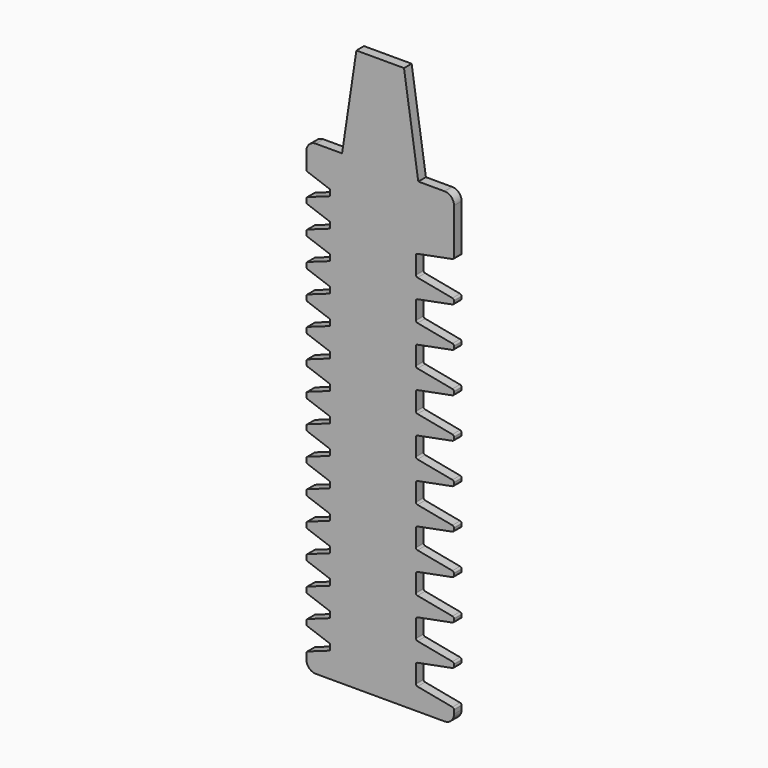
from build123d import *

# Parameters (mm, degrees)
F1_DEPTH  = 0.635
F2_R      = 1.27
F4_DEPTH  = 12.7
F6_DEPTH  = 12.7
F8_DEPTH  = 0.635
F11_DEPTH = 12.7


with BuildPart() as f1:
    # F0 (on Front) → F1 (new body, symmetric)
    with BuildSketch(Plane.XZ):
        Polygon((-9.8425, -12.7), (-9.8425, -62.23), (0, -62.23), (9.8425, -62.23), (9.8425, -12.7), (9.8425, 0), (3.175, 0), (0, 0), (-3.175, 0), (-9.8425, 0), align=None)
        Polygon((-3.175, 12.7), (-3.175, 0), (0, 0), (3.175, 0), (3.175, 12.7), (0, 12.7), align=None)
    extrude(amount=F1_DEPTH, both=True)

    # F2
    f2_edges = [f1.edges().sort_by_distance(p)[0] for p in [
        (9.8425, 0, -62.23),
        (-9.8425, 0, -62.23),
        (-9.8425, 0, 0),
        (9.8425, 0, 0),
    ]]
    fillet(f2_edges, radius=F2_R)

    # F3 (on Front) → F4 (cut, symmetric)
    with BuildSketch(Plane.XZ):
        with BuildLine():
            Line((9.8425, -57.9145550728), (9.8425, -55.3745550728))
            ThreePointArc((9.8425, -55.3745550728), (9.7843008142, -55.536351368), (9.6363736917, -55.6240026818))
            Line((9.6363736917, -55.6240026818), (4.9686263083, -56.5198312683))
            ThreePointArc((4.9686263083, -56.5198312683), (4.8206991858, -56.607482582), (4.7625, -56.7692788773))
            Line((4.7625, -56.7692788773), (4.7625, -57.9145550728))
            Line((4.7625, -57.9145550728), (9.8425, -57.9145550728))
        make_face()
        with BuildLine():
            Line((9.8425, -60.4545550728), (9.8425, -57.9145550728))
            Line((9.8425, -57.9145550728), (4.7625, -57.9145550728))
            Line((4.7625, -57.9145550728), (4.7625, -59.0598312683))
            ThreePointArc((4.7625, -59.0598312683), (4.8206991858, -59.2216275635), (4.9686263083, -59.3092788773))
            Line((4.9686263083, -59.3092788773), (9.6363736917, -60.2051074638))
            ThreePointArc((9.6363736917, -60.2051074638), (9.7843008142, -60.2927587775), (9.8425, -60.4545550728))
        make_face()
    extrude(amount=F4_DEPTH, both=True, mode=Mode.SUBTRACT)

    # F5 (on Front) → F6 (cut, symmetric)
    with BuildSketch(Plane.XZ):
        with BuildLine():
            Line((9.8425, -57.9145550728), (9.8425, -55.3745550728))
            ThreePointArc((9.8425, -55.3745550728), (9.7843008142, -55.536351368), (9.6363736917, -55.6240026818))
            Line((9.6363736917, -55.6240026818), (4.9686263083, -56.5198312683))
            ThreePointArc((4.9686263083, -56.5198312683), (4.8206991858, -56.607482582), (4.7625, -56.7692788773))
            Line((4.7625, -56.7692788773), (4.7625, -57.9145550728))
            Line((4.7625, -57.9145550728), (4.7625, -59.0598312683))
            ThreePointArc((4.7625, -59.0598312683), (4.8206991858, -59.2216275635), (4.9686263083, -59.3092788773))
            Line((4.9686263083, -59.3092788773), (9.6363736917, -60.2051074638))
            ThreePointArc((9.6363736917, -60.2051074638), (9.7843008142, -60.2927587775), (9.8425, -60.4545550728))
            Line((9.8425, -60.4545550728), (9.8425, -57.9145550728))
        make_face()
        with BuildLine():
            Line((9.6363736917, -50.2900026818), (4.9686263083, -51.1858312683))
            ThreePointArc((4.9686263083, -51.1858312683), (4.8206991858, -51.273482582), (4.7625, -51.4352788773))
            Line((4.7625, -51.4352788773), (4.7625, -52.5805550728))
            Line((4.7625, -52.5805550728), (4.7625, -53.7258312683))
            ThreePointArc((4.7625, -53.7258312683), (4.8206991858, -53.8876275635), (4.9686263083, -53.9752788773))
            Line((4.9686263083, -53.9752788773), (9.6363736917, -54.8711074638))
            ThreePointArc((9.6363736917, -54.8711074638), (9.7843008142, -54.9587587775), (9.8425, -55.1205550728))
            Line((9.8425, -55.1205550728), (9.8425, -52.5805550728))
            Line((9.8425, -52.5805550728), (9.8425, -50.0405550728))
            ThreePointArc((9.8425, -50.0405550728), (9.7843008142, -50.202351368), (9.6363736917, -50.2900026818))
        make_face()
        with BuildLine():
            Line((9.6363736917, -44.9560026818), (4.9686263083, -45.8518312683))
            ThreePointArc((4.9686263083, -45.8518312683), (4.8206991858, -45.939482582), (4.7625, -46.1012788773))
            Line((4.7625, -46.1012788773), (4.7625, -47.2465550728))
            Line((4.7625, -47.2465550728), (4.7625, -48.3918312683))
            ThreePointArc((4.7625, -48.3918312683), (4.8206991858, -48.5536275635), (4.9686263083, -48.6412788773))
            Line((4.9686263083, -48.6412788773), (9.6363736917, -49.5371074638))
            ThreePointArc((9.6363736917, -49.5371074638), (9.7843008142, -49.6247587775), (9.8425, -49.7865550728))
            Line((9.8425, -49.7865550728), (9.8425, -47.2465550728))
            Line((9.8425, -47.2465550728), (9.8425, -44.7065550728))
            ThreePointArc((9.8425, -44.7065550728), (9.7843008142, -44.868351368), (9.6363736917, -44.9560026818))
        make_face()
        with BuildLine():
            Line((9.6363736917, -39.6220026818), (4.9686263083, -40.5178312683))
            ThreePointArc((4.9686263083, -40.5178312683), (4.8206991858, -40.605482582), (4.7625, -40.7672788773))
            Line((4.7625, -40.7672788773), (4.7625, -41.9125550728))
            Line((4.7625, -41.9125550728), (4.7625, -43.0578312683))
            ThreePointArc((4.7625, -43.0578312683), (4.8206991858, -43.2196275635), (4.9686263083, -43.3072788773))
            Line((4.9686263083, -43.3072788773), (9.6363736917, -44.2031074638))
            ThreePointArc((9.6363736917, -44.2031074638), (9.7843008142, -44.2907587775), (9.8425, -44.4525550728))
            Line((9.8425, -44.4525550728), (9.8425, -41.9125550728))
            Line((9.8425, -41.9125550728), (9.8425, -39.3725550728))
            ThreePointArc((9.8425, -39.3725550728), (9.7843008142, -39.534351368), (9.6363736917, -39.6220026818))
        make_face()
        with BuildLine():
            Line((9.6363736917, -34.2880026818), (4.9686263083, -35.1838312683))
            ThreePointArc((4.9686263083, -35.1838312683), (4.8206991858, -35.271482582), (4.7625, -35.4332788773))
            Line((4.7625, -35.4332788773), (4.7625, -36.5785550728))
            Line((4.7625, -36.5785550728), (4.7625, -37.7238312683))
            ThreePointArc((4.7625, -37.7238312683), (4.8206991858, -37.8856275635), (4.9686263083, -37.9732788773))
            Line((4.9686263083, -37.9732788773), (9.6363736917, -38.8691074638))
            ThreePointArc((9.6363736917, -38.8691074638), (9.7843008142, -38.9567587775), (9.8425, -39.1185550728))
            Line((9.8425, -39.1185550728), (9.8425, -36.5785550728))
            Line((9.8425, -36.5785550728), (9.8425, -34.0385550728))
            ThreePointArc((9.8425, -34.0385550728), (9.7843008142, -34.200351368), (9.6363736917, -34.2880026818))
        make_face()
        with BuildLine():
            Line((9.6363736917, -28.9540026818), (4.9686263083, -29.8498312683))
            ThreePointArc((4.9686263083, -29.8498312683), (4.8206991858, -29.937482582), (4.7625, -30.0992788773))
            Line((4.7625, -30.0992788773), (4.7625, -31.2445550728))
            Line((4.7625, -31.2445550728), (4.7625, -32.3898312683))
            ThreePointArc((4.7625, -32.3898312683), (4.8206991858, -32.5516275635), (4.9686263083, -32.6392788773))
            Line((4.9686263083, -32.6392788773), (9.6363736917, -33.5351074638))
            ThreePointArc((9.6363736917, -33.5351074638), (9.7843008142, -33.6227587775), (9.8425, -33.7845550728))
            Line((9.8425, -33.7845550728), (9.8425, -31.2445550728))
            Line((9.8425, -31.2445550728), (9.8425, -28.7045550728))
            ThreePointArc((9.8425, -28.7045550728), (9.7843008142, -28.866351368), (9.6363736917, -28.9540026818))
        make_face()
        with BuildLine():
            Line((9.6363736917, -23.6200026818), (4.9686263083, -24.5158312683))
            ThreePointArc((4.9686263083, -24.5158312683), (4.8206991858, -24.603482582), (4.7625, -24.7652788773))
            Line((4.7625, -24.7652788773), (4.7625, -25.9105550728))
            Line((4.7625, -25.9105550728), (4.7625, -27.0558312683))
            ThreePointArc((4.7625, -27.0558312683), (4.8206991858, -27.2176275635), (4.9686263083, -27.3052788773))
            Line((4.9686263083, -27.3052788773), (9.6363736917, -28.2011074638))
            ThreePointArc((9.6363736917, -28.2011074638), (9.7843008142, -28.2887587775), (9.8425, -28.4505550728))
            Line((9.8425, -28.4505550728), (9.8425, -25.9105550728))
            Line((9.8425, -25.9105550728), (9.8425, -23.3705550728))
            ThreePointArc((9.8425, -23.3705550728), (9.7843008142, -23.532351368), (9.6363736917, -23.6200026818))
        make_face()
        with BuildLine():
            Line((9.6363736917, -18.2860026818), (4.9686263083, -19.1818312683))
            ThreePointArc((4.9686263083, -19.1818312683), (4.8206991858, -19.269482582), (4.7625, -19.4312788773))
            Line((4.7625, -19.4312788773), (4.7625, -20.5765550728))
            Line((4.7625, -20.5765550728), (4.7625, -21.7218312683))
            ThreePointArc((4.7625, -21.7218312683), (4.8206991858, -21.8836275635), (4.9686263083, -21.9712788773))
            Line((4.9686263083, -21.9712788773), (9.6363736917, -22.8671074638))
            ThreePointArc((9.6363736917, -22.8671074638), (9.7843008142, -22.9547587775), (9.8425, -23.1165550728))
            Line((9.8425, -23.1165550728), (9.8425, -20.5765550728))
            Line((9.8425, -20.5765550728), (9.8425, -18.0365550728))
            ThreePointArc((9.8425, -18.0365550728), (9.7843008142, -18.198351368), (9.6363736917, -18.2860026818))
        make_face()
        with BuildLine():
            Line((9.6363736917, -12.9520026818), (4.9686263083, -13.8478312683))
            ThreePointArc((4.9686263083, -13.8478312683), (4.8206991858, -13.935482582), (4.7625, -14.0972788773))
            Line((4.7625, -14.0972788773), (4.7625, -15.2425550728))
            Line((4.7625, -15.2425550728), (4.7625, -16.3878312683))
            ThreePointArc((4.7625, -16.3878312683), (4.8206991858, -16.5496275635), (4.9686263083, -16.6372788773))
            Line((4.9686263083, -16.6372788773), (9.6363736917, -17.5331074638))
            ThreePointArc((9.6363736917, -17.5331074638), (9.7843008142, -17.6207587775), (9.8425, -17.7825550728))
            Line((9.8425, -17.7825550728), (9.8425, -15.2425550728))
            Line((9.8425, -15.2425550728), (9.8425, -12.7025550728))
            ThreePointArc((9.8425, -12.7025550728), (9.7843008142, -12.864351368), (9.6363736917, -12.9520026818))
        make_face()
        with BuildLine():
            Line((9.6363736917, -7.6180026818), (4.9686263083, -8.5138312683))
            ThreePointArc((4.9686263083, -8.5138312683), (4.8206991858, -8.601482582), (4.7625, -8.7632788773))
            Line((4.7625, -8.7632788773), (4.7625, -9.9085550728))
            Line((4.7625, -9.9085550728), (4.7625, -11.0538312683))
            ThreePointArc((4.7625, -11.0538312683), (4.8206991858, -11.2156275635), (4.9686263083, -11.3032788773))
            Line((4.9686263083, -11.3032788773), (9.6363736917, -12.1991074638))
            ThreePointArc((9.6363736917, -12.1991074638), (9.7843008142, -12.2867587775), (9.8425, -12.4485550728))
            Line((9.8425, -12.4485550728), (9.8425, -9.9085550728))
            Line((9.8425, -9.9085550728), (9.8425, -7.3685550728))
            ThreePointArc((9.8425, -7.3685550728), (9.7843008142, -7.530351368), (9.6363736917, -7.6180026818))
        make_face()
    extrude(amount=F6_DEPTH, both=True, mode=Mode.SUBTRACT)

    # F7 (on Front) → F8 (join, symmetric)
    with BuildSketch(Plane.XZ):
        Polygon((-3.175, 12.7), (-5.08, 0), (0, 0), (5.08, 0), (3.175, 12.7), align=None)
    extrude(amount=F8_DEPTH, both=True)

    # F10 (on Front) → F11 (cut, symmetric)
    with BuildSketch(Plane.XZ):
        with BuildLine():
            Line((-9.8425, -56.769), (-9.8425, -60.198))
            ThreePointArc((-9.8425, -60.198), (-9.7961774075, -60.0517601476), (-9.6741055557, -59.9588605243))
            Line((-9.6741055557, -59.9588605243), (-6.7943923967, -58.928))
            ThreePointArc((-6.7943923967, -58.928), (-6.7024060494, -58.8579961712), (-6.6675, -58.7477982045))
            Line((-6.6675, -58.7477982045), (-6.6675, -58.2192017955))
            ThreePointArc((-6.6675, -58.2192017955), (-6.7024060494, -58.1090038288), (-6.7943923967, -58.039))
            Line((-6.7943923967, -58.039), (-9.6741055557, -57.0081394757))
            ThreePointArc((-9.6741055557, -57.0081394757), (-9.7961774075, -56.9152398524), (-9.8425, -56.769))
        make_face()
        with BuildLine():
            Line((-9.8425, -52.959), (-9.8425, -56.388))
            ThreePointArc((-9.8425, -56.388), (-9.7961774075, -56.2417601476), (-9.6741055557, -56.1488605243))
            Line((-9.6741055557, -56.1488605243), (-6.7943923967, -55.118))
            ThreePointArc((-6.7943923967, -55.118), (-6.7024060494, -55.0479961712), (-6.6675, -54.9377982045))
            Line((-6.6675, -54.9377982045), (-6.6675, -54.4092017955))
            ThreePointArc((-6.6675, -54.4092017955), (-6.7024060494, -54.2990038288), (-6.7943923967, -54.229))
            Line((-6.7943923967, -54.229), (-9.6741055557, -53.1981394757))
            ThreePointArc((-9.6741055557, -53.1981394757), (-9.7961774075, -53.1052398524), (-9.8425, -52.959))
        make_face()
        with BuildLine():
            Line((-9.8425, -49.149), (-9.8425, -52.578))
            ThreePointArc((-9.8425, -52.578), (-9.7961774075, -52.4317601476), (-9.6741055557, -52.3388605243))
            Line((-9.6741055557, -52.3388605243), (-6.7943923967, -51.308))
            ThreePointArc((-6.7943923967, -51.308), (-6.7024060494, -51.2379961712), (-6.6675, -51.1277982045))
            Line((-6.6675, -51.1277982045), (-6.6675, -50.5992017955))
            ThreePointArc((-6.6675, -50.5992017955), (-6.7024060494, -50.4890038288), (-6.7943923967, -50.419))
            Line((-6.7943923967, -50.419), (-9.6741055557, -49.3881394757))
            ThreePointArc((-9.6741055557, -49.3881394757), (-9.7961774075, -49.2952398524), (-9.8425, -49.149))
        make_face()
        with BuildLine():
            Line((-9.8425, -45.339), (-9.8425, -48.768))
            ThreePointArc((-9.8425, -48.768), (-9.7961774075, -48.6217601476), (-9.6741055557, -48.5288605243))
            Line((-9.6741055557, -48.5288605243), (-6.7943923967, -47.498))
            ThreePointArc((-6.7943923967, -47.498), (-6.7024060494, -47.4279961712), (-6.6675, -47.3177982045))
            Line((-6.6675, -47.3177982045), (-6.6675, -46.7892017955))
            ThreePointArc((-6.6675, -46.7892017955), (-6.7024060494, -46.6790038288), (-6.7943923967, -46.609))
            Line((-6.7943923967, -46.609), (-9.6741055557, -45.5781394757))
            ThreePointArc((-9.6741055557, -45.5781394757), (-9.7961774075, -45.4852398524), (-9.8425, -45.339))
        make_face()
        with BuildLine():
            Line((-9.8425, -41.529), (-9.8425, -44.958))
            ThreePointArc((-9.8425, -44.958), (-9.7961774075, -44.8117601476), (-9.6741055557, -44.7188605243))
            Line((-9.6741055557, -44.7188605243), (-6.7943923967, -43.688))
            ThreePointArc((-6.7943923967, -43.688), (-6.7024060494, -43.6179961712), (-6.6675, -43.5077982045))
            Line((-6.6675, -43.5077982045), (-6.6675, -42.9792017955))
            ThreePointArc((-6.6675, -42.9792017955), (-6.7024060494, -42.8690038288), (-6.7943923967, -42.799))
            Line((-6.7943923967, -42.799), (-9.6741055557, -41.7681394757))
            ThreePointArc((-9.6741055557, -41.7681394757), (-9.7961774075, -41.6752398524), (-9.8425, -41.529))
        make_face()
        with BuildLine():
            Line((-9.8425, -37.719), (-9.8425, -41.148))
            ThreePointArc((-9.8425, -41.148), (-9.7961774075, -41.0017601476), (-9.6741055557, -40.9088605243))
            Line((-9.6741055557, -40.9088605243), (-6.7943923967, -39.878))
            ThreePointArc((-6.7943923967, -39.878), (-6.7024060494, -39.8079961712), (-6.6675, -39.6977982045))
            Line((-6.6675, -39.6977982045), (-6.6675, -39.1692017955))
            ThreePointArc((-6.6675, -39.1692017955), (-6.7024060494, -39.0590038288), (-6.7943923967, -38.989))
            Line((-6.7943923967, -38.989), (-9.6741055557, -37.9581394757))
            ThreePointArc((-9.6741055557, -37.9581394757), (-9.7961774075, -37.8652398524), (-9.8425, -37.719))
        make_face()
        with BuildLine():
            Line((-9.8425, -33.909), (-9.8425, -37.338))
            ThreePointArc((-9.8425, -37.338), (-9.7961774075, -37.1917601476), (-9.6741055557, -37.0988605243))
            Line((-9.6741055557, -37.0988605243), (-6.7943923967, -36.068))
            ThreePointArc((-6.7943923967, -36.068), (-6.7024060494, -35.9979961712), (-6.6675, -35.8877982045))
            Line((-6.6675, -35.8877982045), (-6.6675, -35.3592017955))
            ThreePointArc((-6.6675, -35.3592017955), (-6.7024060494, -35.2490038288), (-6.7943923967, -35.179))
            Line((-6.7943923967, -35.179), (-9.6741055557, -34.1481394757))
            ThreePointArc((-9.6741055557, -34.1481394757), (-9.7961774075, -34.0552398524), (-9.8425, -33.909))
        make_face()
        with BuildLine():
            Line((-9.8425, -30.099), (-9.8425, -33.528))
            ThreePointArc((-9.8425, -33.528), (-9.7961774075, -33.3817601476), (-9.6741055557, -33.2888605243))
            Line((-9.6741055557, -33.2888605243), (-6.7943923967, -32.258))
            ThreePointArc((-6.7943923967, -32.258), (-6.7024060494, -32.1879961712), (-6.6675, -32.0777982045))
            Line((-6.6675, -32.0777982045), (-6.6675, -31.5492017955))
            ThreePointArc((-6.6675, -31.5492017955), (-6.7024060494, -31.4390038288), (-6.7943923967, -31.369))
            Line((-6.7943923967, -31.369), (-9.6741055557, -30.3381394757))
            ThreePointArc((-9.6741055557, -30.3381394757), (-9.7961774075, -30.2452398524), (-9.8425, -30.099))
        make_face()
        with BuildLine():
            Line((-9.8425, -26.289), (-9.8425, -29.718))
            ThreePointArc((-9.8425, -29.718), (-9.7961774075, -29.5717601476), (-9.6741055557, -29.4788605243))
            Line((-9.6741055557, -29.4788605243), (-6.7943923967, -28.448))
            ThreePointArc((-6.7943923967, -28.448), (-6.7024060494, -28.3779961712), (-6.6675, -28.2677982045))
            Line((-6.6675, -28.2677982045), (-6.6675, -27.7392017955))
            ThreePointArc((-6.6675, -27.7392017955), (-6.7024060494, -27.6290038288), (-6.7943923967, -27.559))
            Line((-6.7943923967, -27.559), (-9.6741055557, -26.5281394757))
            ThreePointArc((-9.6741055557, -26.5281394757), (-9.7961774075, -26.4352398524), (-9.8425, -26.289))
        make_face()
        with BuildLine():
            Line((-9.8425, -22.479), (-9.8425, -25.908))
            ThreePointArc((-9.8425, -25.908), (-9.7961774075, -25.7617601476), (-9.6741055557, -25.6688605243))
            Line((-9.6741055557, -25.6688605243), (-6.7943923967, -24.638))
            ThreePointArc((-6.7943923967, -24.638), (-6.7024060494, -24.5679961712), (-6.6675, -24.4577982045))
            Line((-6.6675, -24.4577982045), (-6.6675, -23.9292017955))
            ThreePointArc((-6.6675, -23.9292017955), (-6.7024060494, -23.8190038288), (-6.7943923967, -23.749))
            Line((-6.7943923967, -23.749), (-9.6741055557, -22.7181394757))
            ThreePointArc((-9.6741055557, -22.7181394757), (-9.7961774075, -22.6252398524), (-9.8425, -22.479))
        make_face()
        with BuildLine():
            Line((-9.8425, -18.669), (-9.8425, -22.098))
            ThreePointArc((-9.8425, -22.098), (-9.7961774075, -21.9517601476), (-9.6741055557, -21.8588605243))
            Line((-9.6741055557, -21.8588605243), (-6.7943923967, -20.828))
            ThreePointArc((-6.7943923967, -20.828), (-6.7024060494, -20.7579961712), (-6.6675, -20.6477982045))
            Line((-6.6675, -20.6477982045), (-6.6675, -20.1192017955))
            ThreePointArc((-6.6675, -20.1192017955), (-6.7024060494, -20.0090038288), (-6.7943923967, -19.939))
            Line((-6.7943923967, -19.939), (-9.6741055557, -18.9081394757))
            ThreePointArc((-9.6741055557, -18.9081394757), (-9.7961774075, -18.8152398524), (-9.8425, -18.669))
        make_face()
        with BuildLine():
            Line((-9.8425, -14.859), (-9.8425, -18.288))
            ThreePointArc((-9.8425, -18.288), (-9.7961774075, -18.1417601476), (-9.6741055557, -18.0488605243))
            Line((-9.6741055557, -18.0488605243), (-6.7943923967, -17.018))
            ThreePointArc((-6.7943923967, -17.018), (-6.7024060494, -16.9479961712), (-6.6675, -16.8377982045))
            Line((-6.6675, -16.8377982045), (-6.6675, -16.3092017955))
            ThreePointArc((-6.6675, -16.3092017955), (-6.7024060494, -16.1990038288), (-6.7943923967, -16.129))
            Line((-6.7943923967, -16.129), (-9.6741055557, -15.0981394757))
            ThreePointArc((-9.6741055557, -15.0981394757), (-9.7961774075, -15.0052398524), (-9.8425, -14.859))
        make_face()
        with BuildLine():
            Line((-9.8425, -11.049), (-9.8425, -14.478))
            ThreePointArc((-9.8425, -14.478), (-9.7961774075, -14.3317601476), (-9.6741055557, -14.2388605243))
            Line((-9.6741055557, -14.2388605243), (-6.7943923967, -13.208))
            ThreePointArc((-6.7943923967, -13.208), (-6.7024060494, -13.1379961712), (-6.6675, -13.0277982045))
            Line((-6.6675, -13.0277982045), (-6.6675, -12.4992017955))
            ThreePointArc((-6.6675, -12.4992017955), (-6.7024060494, -12.3890038288), (-6.7943923967, -12.319))
            Line((-6.7943923967, -12.319), (-9.6741055557, -11.2881394757))
            ThreePointArc((-9.6741055557, -11.2881394757), (-9.7961774075, -11.1952398524), (-9.8425, -11.049))
        make_face()
        with BuildLine():
            Line((-9.8425, -7.239), (-9.8425, -10.668))
            ThreePointArc((-9.8425, -10.668), (-9.7961774075, -10.5217601476), (-9.6741055557, -10.4288605243))
            Line((-9.6741055557, -10.4288605243), (-6.7943923967, -9.398))
            ThreePointArc((-6.7943923967, -9.398), (-6.7024060494, -9.3279961712), (-6.6675, -9.2177982045))
            Line((-6.6675, -9.2177982045), (-6.6675, -8.6892017955))
            ThreePointArc((-6.6675, -8.6892017955), (-6.7024060494, -8.5790038288), (-6.7943923967, -8.509))
            Line((-6.7943923967, -8.509), (-9.6741055557, -7.4781394757))
            ThreePointArc((-9.6741055557, -7.4781394757), (-9.7961774075, -7.3852398524), (-9.8425, -7.239))
        make_face()
        with BuildLine():
            Line((-9.8425, -3.429), (-9.8425, -6.858))
            ThreePointArc((-9.8425, -6.858), (-9.7961774075, -6.7117601476), (-9.6741055557, -6.6188605243))
            Line((-9.6741055557, -6.6188605243), (-6.7943923967, -5.588))
            ThreePointArc((-6.7943923967, -5.588), (-6.7024060494, -5.5179961712), (-6.6675, -5.4077982045))
            Line((-6.6675, -5.4077982045), (-6.6675, -4.8792017955))
            ThreePointArc((-6.6675, -4.8792017955), (-6.7024060494, -4.7690038288), (-6.7943923967, -4.699))
            Line((-6.7943923967, -4.699), (-9.6741055557, -3.6681394757))
            ThreePointArc((-9.6741055557, -3.6681394757), (-9.7961774075, -3.5752398524), (-9.8425, -3.429))
        make_face()
    extrude(amount=F11_DEPTH, both=True, mode=Mode.SUBTRACT)


solid = f1.part
